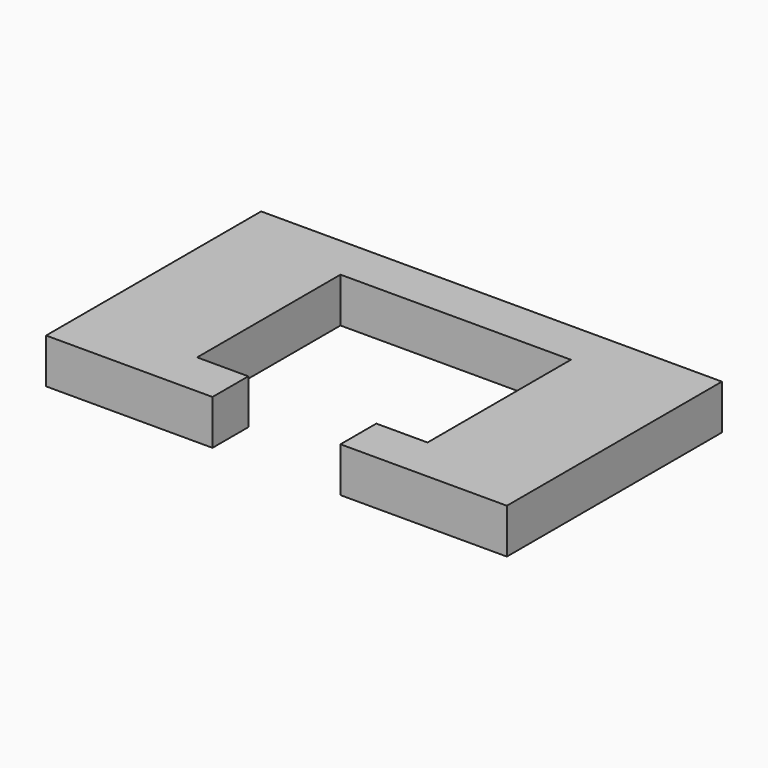
from build123d import *

# Parameters (mm, degrees)
F1_DEPTH = 7


# Not quite as in the source:
# - ends of sketch curves that miss each other by under 0.0002 mm in the source are joined


with BuildPart() as f1:
    # F0 (on Top) → F1 (new body)
    with BuildSketch(Plane.XY):
        Polygon((10, -21), (36, -21), (36, 21), (-36, 21), (-36, -21), (-10, -21), (-10, -13.9999815226), (-18, -14), (-18, 14), (18, 14), (18, -14), (10, -14), align=None)
    extrude(amount=F1_DEPTH)


solid = f1.part
